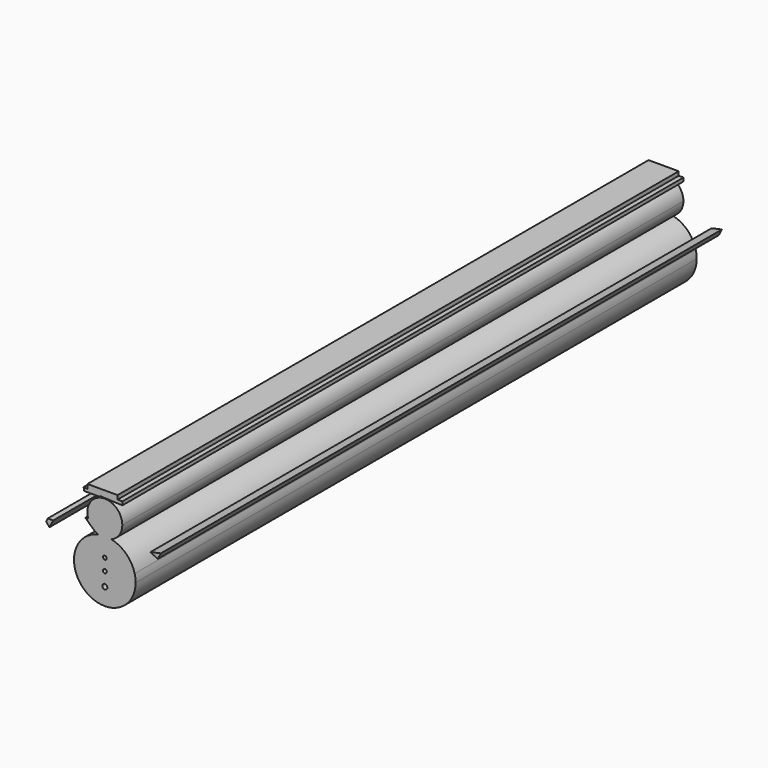
from build123d import *

# Parameters (mm, degrees)
F0_R     = 3.559087352
F0_R_2   = 2.7679837305
F0_R_3   = 2.6213351788
F0_R_4   = 8.8899955153
F0_R_5   = 9.1287938565
F1_DEPTH = 1000


with BuildPart() as f1:
    # F0 (on Front) → F1 (new body)
    with BuildSketch(Plane.XZ):
        with BuildLine():
            ThreePointArc((-42.522289517, -13.1209784431), (-5.5598010496, -67.7275202598), (43.929604165, -24.1511650383))
            ThreePointArc((43.929604165, -24.1511650383), (43.5884245631, -18.6867925953), (42.5701853055, -13.3072983317))
            ThreePointArc((42.5701853055, -13.3072983317), (30.478272359, 7.485602118), (9.2489418796, 18.7937670981))
            ThreePointArc((9.2489418796, 18.7937670981), (0, 17.0136591141), (-9.2489418796, 18.7937670981))
            ThreePointArc((-9.2489418796, 18.7937670981), (-30.4089270744, 7.552261847), (-42.522289517, -13.1209784431))
        make_face()
        with Locations((0, -43.709166348)):
            Circle(F0_R, mode=Mode.SUBTRACT)
        with Locations((0, -24.1511650383)):
            Circle(F0_R_2, mode=Mode.SUBTRACT)
        with Locations((0, -7.2601665743)):
            Circle(F0_R_3, mode=Mode.SUBTRACT)
        with BuildLine():
            ThreePointArc((-9.2489418796, 18.7937670981), (0, 17.0136591141), (9.2489418796, 18.7937670981))
            ThreePointArc((9.2489418796, 18.7937670981), (0, 19.7784391267), (-9.2489418796, 18.7937670981))
        make_face()
        with BuildLine():
            ThreePointArc((-9.2489418796, 18.7937670981), (0, 19.7784391267), (9.2489418796, 18.7937670981))
            ThreePointArc((9.2489418796, 18.7937670981), (20.6318054946, 27.9593809067), (24.9175081308, 41.9311672449))
            ThreePointArc((24.9175081308, 41.9311672449), (17.6193389695, 59.5505062144), (0, 66.8486753757))
            ThreePointArc((0, 66.8486753757), (-20.2470624636, 56.4548951769), (-23.6029080517, 33.9446196208))
            Line((-23.6029080517, 33.9446196208), (-3.51480454, 33.9446196208))
            Line((-3.51480454, 33.9446196208), (-11.8889665349, 30.1777279181))
            Line((-11.8889665349, 30.1777279181), (-19.6945457834, 26.6665978821))
            ThreePointArc((-19.6945457834, 26.6665978821), (-14.9975576566, 22.0325372472), (-9.2489418796, 18.7937670981))
        make_face()
        with Locations((-9.0381670743, 46.3761650026)):
            Circle(F0_R_4, mode=Mode.SUBTRACT)
        with Locations((10.519833304, 46.3761650026)):
            Circle(F0_R_5, mode=Mode.SUBTRACT)
        with BuildLine():
            Line((-19.9842423259, 26.5362856785), (-19.6945457834, 26.6665978821))
            ThreePointArc((-19.6945457834, 26.6665978821), (-21.9524435373, 30.1425102311), (-23.6029080517, 33.9446196208))
            Line((-23.6029080517, 33.9446196208), (-27.814138809, 33.9446196208))
            Line((-27.814138809, 33.9446196208), (-19.9842423259, 26.5362856785))
        make_face()
        with BuildLine():
            ThreePointArc((-23.6029080517, 33.9446196208), (-21.9524435373, 30.1425102311), (-19.6945457834, 26.6665978821))
            Line((-19.6945457834, 26.6665978821), (-11.8889665349, 30.1777279181))
            Line((-11.8889665349, 30.1777279181), (-3.51480454, 33.9446196208))
            Line((-3.51480454, 33.9446196208), (-23.6029080517, 33.9446196208))
        make_face()
        with Locations((-9.0381670743, 46.3761650026)):
            Circle(F0_R_4)
        with Locations((10.519833304, 46.3761650026)):
            Circle(F0_R_5)
    extrude(amount=F1_DEPTH)


with BuildPart() as f1b:
    # F0 (on Front) → F1, piece 2 (new body)
    with BuildSketch(Plane.XZ):
        Polygon((-78.868268081, 5.2594794789), (-76.0095044971, 10.8161661774), (-83.7513430484, 10.8161661774), align=None)
        Polygon((-83.7513430484, 10.8161661774), (-76.0095044971, 10.8161661774), (-73.5702174304, 15.5575005338), (-81.3435018063, 15.5575005338), align=None)
    extrude(amount=F1_DEPTH)


with BuildPart() as f1c:
    # F0 (on Front) → F1, piece 3 (new body)
    with BuildSketch(Plane.XZ):
        Polygon((-29.4851679355, 66.8486753757), (-7.8528337181, 66.8486753757), (-6.3352061266, 67.9107309461), (25.0401664525, 66.5325298905), (25.0401664525, 71.5367647941), (18.2245001197, 71.5367647941), (18.2245001197, 77.201411128), (-24.7861540662, 77.201411128), (-24.7861540662, 70.7344174598), (-30.2779826288, 71.5367647941), align=None)
    extrude(amount=F1_DEPTH)


with BuildPart() as f1d:
    # F0 (on Front) → F1, piece 4 (new body)
    with BuildSketch(Plane.XZ):
        Polygon((65.045170486, 20.8934377879), (75.4168331623, 15.5575005338), (79.8404374607, 24.1558272027), align=None)
    extrude(amount=F1_DEPTH)


solid = Compound([f1.part, f1b.part, f1c.part, f1d.part])
